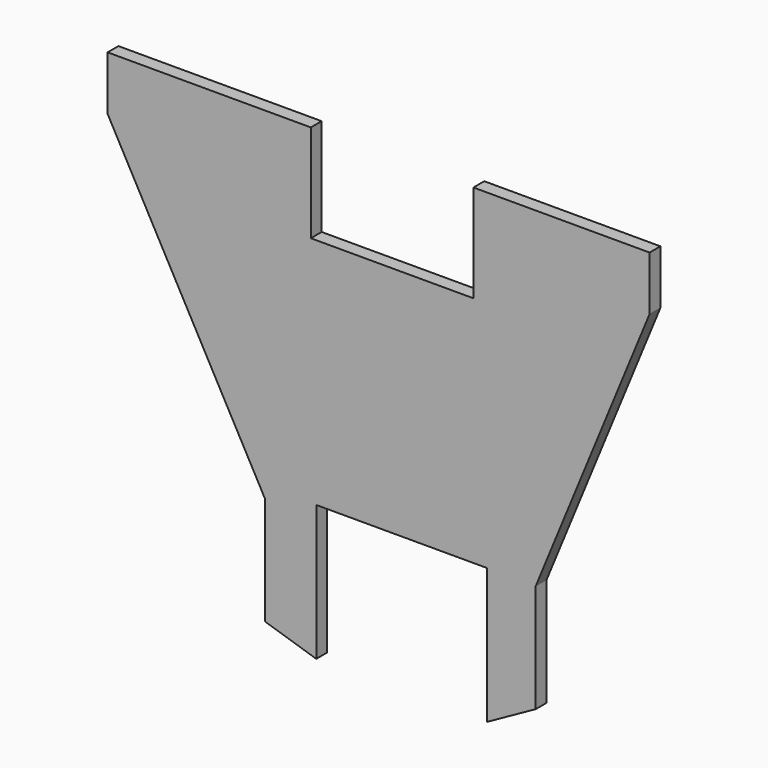
from build123d import *

# Parameters (mm, degrees)
F1_DEPTH = 2.5


# Not quite as in the source:
# - a feature names something its author has since deleted; it is built from what else it names


with BuildPart() as f1:
    # F0 (on Front) → F1 (new body, symmetric)
    with BuildSketch(Plane.XZ):
        Polygon((92, 102), (92, 122), (27, 122), (27, 86), (-33, 86), (-33, 122), (-108, 122), (-108, 102), (-50, -4), (-50, -44), (-31, -50), (-31, 0), (0, 0), (32, 0), (32, -50), (49.9996958359, -40.0000051003), (49.9996958359, -5.1003e-06), align=None)
    extrude(amount=F1_DEPTH, both=True)


solid = f1.part
